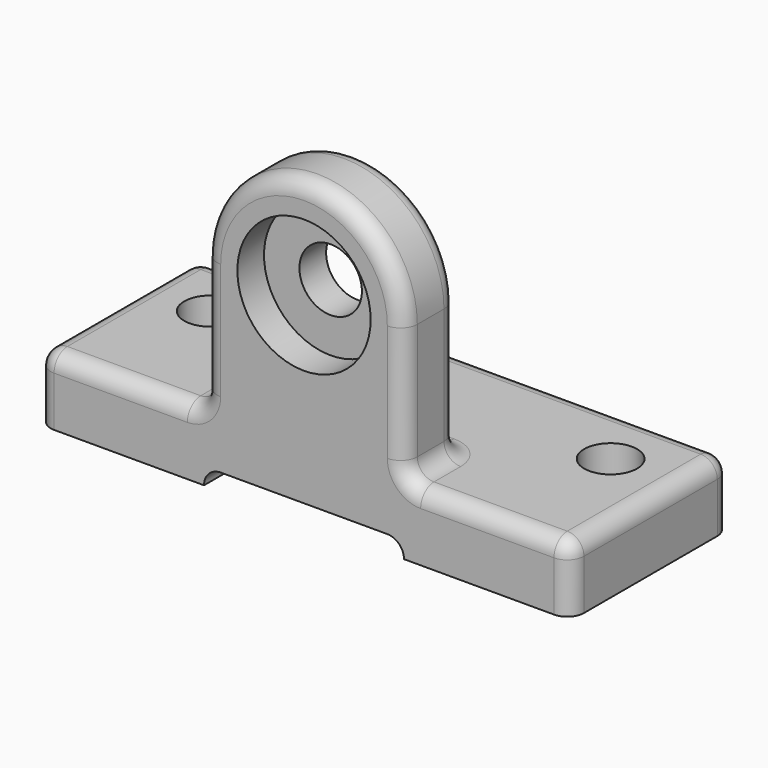
from build123d import *

# Parameters (mm, degrees)
F0_W           = 101.6
F0_H           = 38.1
F1_DEPTH       = 12.7
F2_W           = 38.1
F2_H           = 12.7
F3_DEPTH       = 12.7
F4_D           = 11.90625
F4_CBORE_D     = 25.4
F4_CBORE_DEPTH = 6.35
F5_W           = 38.1
F5_H           = 3.175
F6_DEPTH       = 38.101
F8_D           = 10.0838
F9_D           = 10.0838
F10_R          = 3.175
F11_R          = 3.175
F12_R          = 3.17499


# Not quite as in the source:
# - a fillet or chamfer is up to 0.001 mm smaller than in the source, because OpenCascade refuses the exact size
# - a length typed as a fraction of an inch, garbled in the dataset ("3 / 203.2 mm" for 3/8 in), is restored


with BuildPart() as f1:
    # F0 (on Top) → F1 (new body)
    with BuildSketch(Plane.XY):
        with Locations((50.8, 19.05)):
            Rectangle(F0_W, F0_H)
    extrude(amount=F1_DEPTH)

    # F2 (on face) → F3 (join)
    with BuildSketch(Plane.XZ):
        with BuildLine():
            Line((31.75, 38.1), (31.75, 12.7))
            Line((31.75, 12.7), (69.85, 12.7))
            Line((69.85, 12.7), (69.85, 38.1))
            ThreePointArc((69.85, 38.1), (50.8, 57.15), (31.75, 38.1))
        make_face()
        with Locations((50.8, 6.35)):
            Rectangle(F2_W, F2_H)
    extrude(amount=-F3_DEPTH)

    # F4 (through all)
    with Locations(Plane.XZ):
        with Locations((50.8, 38.1)):
            CounterBoreHole(F4_D / 2, F4_CBORE_D / 2, F4_CBORE_DEPTH)

    # F5 (on face) → F6 (cut, through all)
    with BuildSketch(Plane.XZ):
        with Locations((50.8, 1.5875)):
            Rectangle(F5_W, F5_H)
    extrude(amount=-F6_DEPTH, mode=Mode.SUBTRACT)

    # F8 (through all)
    with Locations(Plane.XY.offset(12.7)):
        with Locations((12.7, 25.4)):
            Hole(F8_D / 2)

    # F9 (through all)
    with Locations(Plane.XY.offset(12.7)):
        with Locations((88.9, 25.4)):
            Hole(F9_D / 2)

    # F10
    f10_edges = [f1.edges().sort_by_distance(p)[0] for p in [
        (101.6, 0, 6.35),
        (0, 0, 6.35),
        (0, 38.1, 6.35),
        (101.6, 38.1, 6.35),
    ]]
    fillet(f10_edges, radius=F10_R)

    # F11
    f11_edges = [f1.edges().sort_by_distance(p)[0] for p in [
        (69.85, 12.7, 25.4),
        (50.8, 12.7, 57.15),
        (31.75, 12.7, 25.4),
        (50.8, 12.7, 12.7),
        (17.4625, 0, 12.7),
        (50.8, 38.1, 12.7),
        (0, 19.05, 12.7),
        (101.6, 19.05, 12.7),
        (84.1375, 0, 12.7),
        (69.85, 0, 25.4),
        (31.75, 0, 25.4),
        (50.8, 0, 57.15),
        (31.75, 6.35, 12.7),
        (69.85, 6.35, 12.7),
        (0.929936, 37.170064, 12.7),
        (0.929936, 0.929936, 12.7),
        (100.670064, 37.170064, 12.7),
    ]]
    fillet(f11_edges, radius=F11_R)

    # F12 (radius 3.175 in the source; OpenCascade refuses exactly that, so slightly less here)
    f12_edges = [f1.edges().sort_by_distance(p)[0] for p in [
        (31.75, 19.05, 3.175),
        (69.85, 19.05, 3.175),
    ]]
    fillet(f12_edges, radius=F12_R)


solid = f1.part
